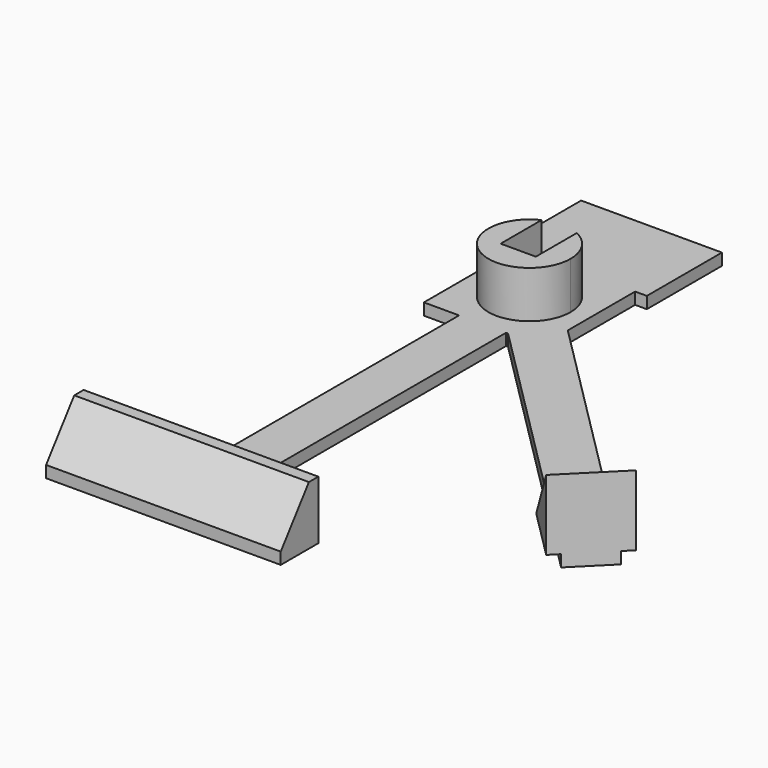
from build123d import *

# Parameters (mm, degrees)
F0_W          = 10
F0_H          = 150
F0_W_2        = 15
F0_H_2        = 31
F1_DEPTH      = 5
F2_DEPTH      = 25
F3_DEPTH      = 25
F5_DEPTH      = 25
F5_DEPTH_BACK = 5
F7_DEPTH      = 100


# Not quite as in the source:
# - a feature names something its author has since deleted; it is built from what else it names


with BuildPart() as f1:
    # F0 (on Top) → F1 (new body)
    with BuildSketch(Plane.XY):
        with BuildLine():
            Line((-70.3635856962, -3.0238344104), (-87.8635856962, -3.0238344104))
            Line((-87.8635856962, -3.0238344104), (-87.8635856962, -53.0238344104))
            Line((-87.8635856962, -53.0238344104), (-72.8635856962, -53.0238344104))
            Line((-72.8635856962, -53.0238344104), (-62.8635856962, -53.0238344104))
            Line((-62.8635856962, -53.0238344104), (-52.8635856962, -53.0238344104))
            Line((-52.8635856962, -53.0238344104), (-52.0057213199, -53.0238344104))
            Line((-52.0057213199, -53.0238344104), (-37.8635856962, -38.8816987866))
            Line((-37.8635856962, -38.8816987866), (-37.8635856962, -3.0238344104))
            Line((-37.8635856962, -3.0238344104), (-55.3635856962, -3.0238344104))
            Line((-55.3635856962, -3.0238344104), (-55.3635856962, -12.2124461095))
            ThreePointArc((-55.3635856962, -12.2124461095), (-48.0733862384, -18.6696909434), (-45.3635856962, -28.0238344104))
            ThreePointArc((-45.3635856962, -28.0238344104), (-72.2177291631, -42.8140338681), (-70.3635856962, -12.2124461095))
            Line((-70.3635856962, -12.2124461095), (-70.3635856962, -3.0238344104))
        make_face()
        with Locations((-67.8635856962, -128.0238344104)):
            Rectangle(F0_W, F0_H)
        with Locations((-57.8635856962, -128.0238344104)):
            Rectangle(F0_W, F0_H)
        Polygon((-37.8635856962, -53.0238344104), (-37.8635856962, -38.8816987866), (-52.0057213199, -53.0238344104), align=None)
        Polygon((75.2734992937, -152.0187837765), (-37.8635856962, -38.8816987866), (-37.8635856962, -53.0238344104), (-52.0057213199, -53.0238344104), (61.13136367, -166.1609194002), align=None)
        Polygon((-92.8635856962, -3.0238344104), (-87.8635856962, -3.0238344104), (-70.3635856962, -3.0238344104), (-70.3635856962, 27.9761655896), (-55.3635856962, 27.9761655896), (-55.3635856962, -3.0238344104), (-37.8635856962, -3.0238344104), (-32.8635856962, -3.0238344104), (-32.8635856962, 36.9761655896), (-92.8635856962, 36.9761655896), align=None)
        with Locations((-62.8635856962, 12.4761655896)):
            Rectangle(F0_W_2, F0_H_2)
        with BuildLine():
            Line((-55.3635856962, -3.0238344104), (-70.3635856962, -3.0238344104))
            Line((-70.3635856962, -3.0238344104), (-70.3635856962, -12.2124461095))
            ThreePointArc((-70.3635856962, -12.2124461095), (-62.8635856962, -10.5238344104), (-55.3635856962, -12.2124461095))
            Line((-55.3635856962, -12.2124461095), (-55.3635856962, -3.0238344104))
        make_face()
        with BuildLine():
            ThreePointArc((-55.3635856962, -12.2124461095), (-62.8635856962, -10.5238344104), (-70.3635856962, -12.2124461095))
            Line((-70.3635856962, -12.2124461095), (-70.3635856962, -34.0238344104))
            Line((-70.3635856962, -34.0238344104), (-55.3635856962, -34.0238344104))
            Line((-55.3635856962, -34.0238344104), (-55.3635856962, -12.2124461095))
        make_face()
    extrude(amount=F1_DEPTH)

    # F0 (on Top) → F2 (join)
    with BuildSketch(Plane.XY):
        with BuildLine():
            Line((-70.3635856962, -34.0238344104), (-70.3635856962, -12.2124461095))
            ThreePointArc((-70.3635856962, -12.2124461095), (-72.2177291631, -42.8140338681), (-45.3635856962, -28.0238344104))
            ThreePointArc((-45.3635856962, -28.0238344104), (-48.0733862384, -18.6696909434), (-55.3635856962, -12.2124461095))
            Line((-55.3635856962, -12.2124461095), (-55.3635856962, -34.0238344104))
            Line((-55.3635856962, -34.0238344104), (-70.3635856962, -34.0238344104))
        make_face()
    extrude(amount=F2_DEPTH)

    # F0 (on Top) → F3 (join)
    with BuildSketch(Plane.XY):
        Polygon((-62.8635856962, -203.0238344104), (-72.8635856962, -203.0238344104), (-112.8635856962, -203.0238344104), (-112.8635856962, -223.0238344104), (-12.8635856962, -223.0238344104), (-12.8635856962, -203.0238344104), (-52.8635856962, -203.0238344104), align=None)
    extrude(amount=F3_DEPTH)

    # F4 (on face) → F5 (join, two sides)
    with BuildSketch(Plane(origin=(-38.3726422414, -38.3726422414, 0), x_dir=(-0.7071067812, 0.7071067812, 0), z_dir=(0.7071067812, 0.7071067812, 0))) as f5_sk:
        Polygon((-160.7199146703, 35), (-160.7199146703, 5), (-130.7199146703, 5), align=None)
    extrude(amount=-F5_DEPTH)
    extrude(f5_sk.sketch, amount=F5_DEPTH_BACK)

    # F6 (on face) → F7 (cut, through all)
    with BuildSketch(Plane(origin=(-112.8635856962, 0, 0), x_dir=(0, -1, 0), z_dir=(-1, 0, 0))):
        Polygon((223.0238344104, 25), (208.0238344104, 25), (223.0238344104, 5), align=None)
    extrude(amount=-F7_DEPTH, mode=Mode.SUBTRACT)


solid = f1.part
